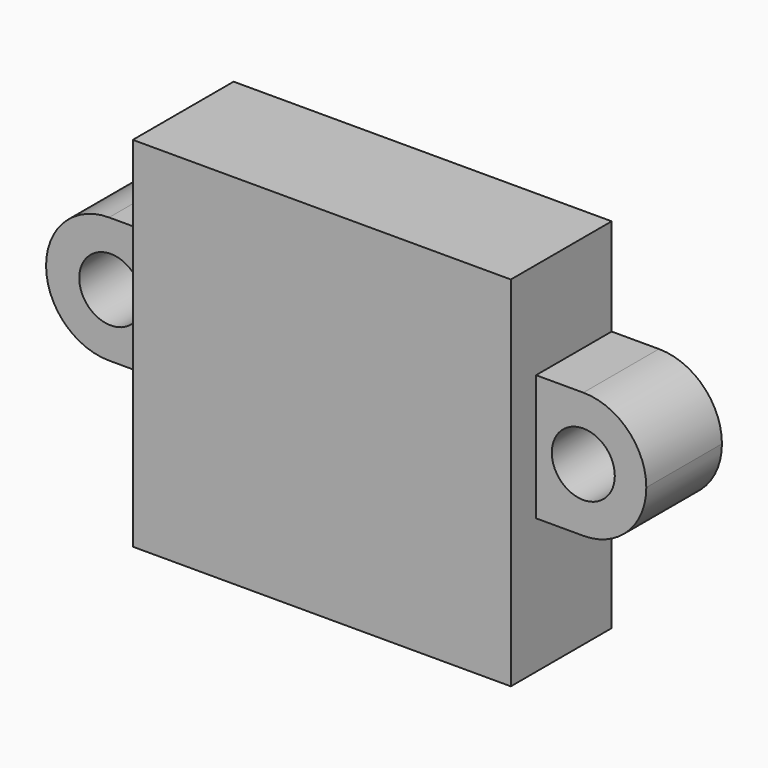
from build123d import *

# Parameters (mm, degrees)
F0_W     = 20
F0_H     = 20
F0_R     = 1.75
F1_DEPTH = 2
F0_R_2   = 2
F2_DEPTH = 6


# Not quite as in the source:
# - a feature names something its author has since deleted; it is built from what else it names


with BuildPart() as f1:
    # F0 (on Front) → F1 (new body)
    with BuildSketch(Plane.XZ):
        Polygon((-29.00025, 5.7325412996), (-29.00025, 25.7325412996), (-9.00025, 25.7325412996), (-9.00025, 5.7325412996), (-7.00025, 5.7325412996), (-7.00025, 14.311070554), (-7.00025, 22.311070554), (-7.00025, 28.4722108253), (-31.00025, 28.4722108253), (-31.00025, 22.311070554), (-31.00025, 14.311070554), (-31.00025, 5.7325412996), align=None)
        with Locations((-19.00025, 15.7325412996)):
            Rectangle(F0_W, F0_H)
        with Locations((-19.00025, 15.7325412996)):
            Circle(F0_R, mode=Mode.SUBTRACT)
        with Locations((-19.00025, 15.7325412996)):
            Circle(F0_R)
    extrude(amount=F1_DEPTH)

    # F0 (on Front) → F2 (join)
    with BuildSketch(Plane.XZ):
        Polygon((-29.00025, 5.7325412996), (-29.00025, 25.7325412996), (-9.00025, 25.7325412996), (-9.00025, 5.7325412996), (-7.00025, 5.7325412996), (-7.00025, 14.311070554), (-7.00025, 22.311070554), (-7.00025, 28.4722108253), (-31.00025, 28.4722108253), (-31.00025, 22.311070554), (-31.00025, 14.311070554), (-31.00025, 5.7325412996), align=None)
        with BuildLine():
            Line((-7.00025, 22.311070554), (-7.00025, 14.311070554))
            Line((-7.00025, 14.311070554), (-4, 14.311070554))
            ThreePointArc((-4, 14.311070554), (-1.1715728753, 15.4826434292), (0, 18.311070554))
            ThreePointArc((0, 18.311070554), (-1.1715728753, 21.1394976787), (-4, 22.311070554))
            Line((-4, 22.311070554), (-7.00025, 22.311070554))
        make_face()
        with Locations((-4, 18.311070554)):
            Circle(F0_R_2, mode=Mode.SUBTRACT)
        with Locations((-19.00025, 15.7325412996)):
            Circle(F0_R)
        with BuildLine():
            Line((-34.1055206901, 14.311070554), (-31.00025, 14.311070554))
            Line((-31.00025, 14.311070554), (-31.00025, 22.311070554))
            Line((-31.00025, 22.311070554), (-34.1055206901, 22.311070554))
            ThreePointArc((-34.1055206901, 22.311070554), (-38.1055206901, 18.311070554), (-34.1055206901, 14.311070554))
        make_face()
        with Locations((-34, 18.311070554)):
            Circle(F0_R_2, mode=Mode.SUBTRACT)
    extrude(amount=-F2_DEPTH)


solid = f1.part
